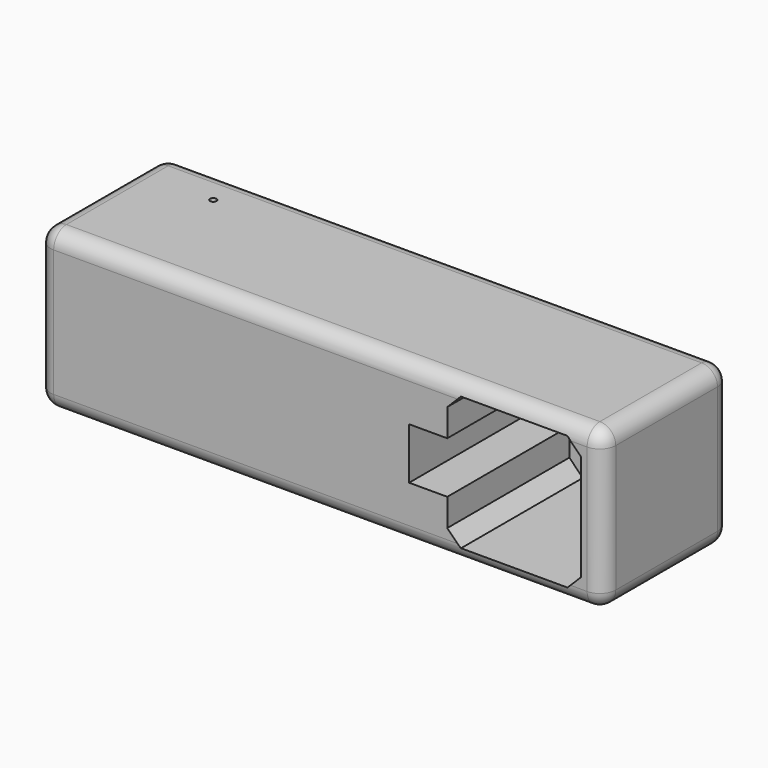
from build123d import *

# Parameters (mm, degrees)
F0_W           = 177.8
F0_H           = 50
F1_DEPTH       = 50
F2_W           = 12
F2_H           = 16.2
F3_DEPTH       = 50
F4_R           = 11
F5_DEPTH       = 5
F7_DEPTH       = 15
F8_R           = 0.49999
F9_T1_DEPTH    = 40
F9_T3_DEPTH    = 167.8
F9_T5_DEPTH    = 40
F9_S9_W        = 5
F9_S9_H        = 5
F9_T10_DEPTH   = 5
F9_S15_W       = 5
F9_S15_H       = 5
F9_T16_DEPTH   = 5
F9_S21_W       = 5
F9_S21_H       = 5
F9_T22_DEPTH   = 5
F9_S27_W       = 5
F9_S27_H       = 5
F9_T28_DEPTH   = 5
F9_S33_W       = 5
F9_S33_H       = 5
F9_T34_DEPTH   = 5
F9_S39_W       = 5
F9_S39_H       = 5
F9_T40_DEPTH   = 5
F9_S45_W       = 5
F9_S45_H       = 5
F9_T46_DEPTH   = 5
F9_S51_W       = 5
F9_S51_H       = 5
F9_T52_DEPTH   = 5
F10_R          = 1.6
F11_DEPTH      = 1
F12_R          = 1
F13_DEPTH      = 2
F13_DEPTH_BACK = 1
F14_DEPTH      = 25
F15_DEPTH      = 2
F16_R          = 11
F17_DEPTH      = 25


# Not quite as in the source:
# - a fillet or chamfer that OpenCascade refuses, or shapes differently, is made with other operations: its cross-section is extruded or revolved along the edge and cut away or added
# - a fillet or chamfer is up to 0.001 mm smaller than in the source, because OpenCascade refuses the exact size


with BuildPart() as f1:
    # F0 (on Front) → F1 (new body)
    with BuildSketch(Plane.XZ):
        Rectangle(F0_W, F0_H)
    extrude(amount=F1_DEPTH)

    # F2 (on face) → F3 (cut, through all)
    with BuildSketch(Plane(origin=(0, 0, 0), x_dir=(-1, 0, 0), z_dir=(0, 1, 0))):
        Polygon((-44.1426406871, 21), (-77.6573593129, 21), (-81.9, 16.7573593129), (-81.9, -16.7573593129), (-77.6573593129, -21), (-44.1426406871, -21), (-39.9, -16.7573593129), (-39.9, -8.1), (-39.9, 8.1), (-39.9, 16.7573593129), align=None)
        with BuildLine():
            ThreePointArc((-75, -15.6), (-77.5606601718, -16.6606601718), (-76.5, -14.1))
            Line((-76.5, -14.1), (-76.5, 14.1))
            ThreePointArc((-76.5, 14.1), (-77.5606601718, 16.6606601718), (-75, 15.6))
            Line((-75, 15.6), (-46.8, 15.6))
            ThreePointArc((-46.8, 15.6), (-45.3, 17.1), (-43.8, 15.6))
            ThreePointArc((-43.8, 15.6), (-44.2393398282, 14.5393398282), (-45.3, 14.1))
            Line((-45.3, 14.1), (-45.3, -14.1))
            ThreePointArc((-45.3, -14.1), (-44.2393398282, -14.5393398282), (-43.8, -15.6))
            ThreePointArc((-43.8, -15.6), (-45.3, -17.1), (-46.8, -15.6))
            Line((-46.8, -15.6), (-75, -15.6))
        make_face(mode=Mode.SUBTRACT)
        with Locations((-33.9, 0)):
            Rectangle(F2_W, F2_H)
        with BuildLine():
            Line((-75, -15.6), (-76.5, -15.6))
            Line((-76.5, -15.6), (-76.5, -14.1))
            ThreePointArc((-76.5, -14.1), (-77.5606601718, -16.6606601718), (-75, -15.6))
        make_face()
        with BuildLine():
            Line((-76.5, -14.1), (-76.5, -15.6))
            Line((-76.5, -15.6), (-75, -15.6))
            ThreePointArc((-75, -15.6), (-75.4393398282, -14.5393398282), (-76.5, -14.1))
        make_face()
        with BuildLine():
            Line((-76.5, 14.1), (-76.5, -14.1))
            ThreePointArc((-76.5, -14.1), (-75.4393398282, -14.5393398282), (-75, -15.6))
            Line((-75, -15.6), (-46.8, -15.6))
            ThreePointArc((-46.8, -15.6), (-46.3606601718, -14.5393398282), (-45.3, -14.1))
            Line((-45.3, -14.1), (-45.3, 14.1))
            ThreePointArc((-45.3, 14.1), (-46.3606601718, 14.5393398282), (-46.8, 15.6))
            Line((-46.8, 15.6), (-75, 15.6))
            ThreePointArc((-75, 15.6), (-75.4393398282, 14.5393398282), (-76.5, 14.1))
        make_face()
        with BuildLine():
            ThreePointArc((-75, 15.6), (-77.5606601718, 16.6606601718), (-76.5, 14.1))
            Line((-76.5, 14.1), (-76.5, 15.6))
            Line((-76.5, 15.6), (-75, 15.6))
        make_face()
        with BuildLine():
            Line((-76.5, 15.6), (-76.5, 14.1))
            ThreePointArc((-76.5, 14.1), (-75.4393398282, 14.5393398282), (-75, 15.6))
            Line((-75, 15.6), (-76.5, 15.6))
        make_face()
        with BuildLine():
            ThreePointArc((-45.3, -14.1), (-46.3606601718, -14.5393398282), (-46.8, -15.6))
            Line((-46.8, -15.6), (-45.3, -15.6))
            Line((-45.3, -15.6), (-45.3, -14.1))
        make_face()
        with BuildLine():
            Line((-45.3, -15.6), (-46.8, -15.6))
            ThreePointArc((-46.8, -15.6), (-45.3, -17.1), (-43.8, -15.6))
            ThreePointArc((-43.8, -15.6), (-44.2393398282, -14.5393398282), (-45.3, -14.1))
            Line((-45.3, -14.1), (-45.3, -15.6))
        make_face()
        with BuildLine():
            ThreePointArc((-43.8, 15.6), (-45.3, 17.1), (-46.8, 15.6))
            Line((-46.8, 15.6), (-45.3, 15.6))
            Line((-45.3, 15.6), (-45.3, 14.1))
            ThreePointArc((-45.3, 14.1), (-44.2393398282, 14.5393398282), (-43.8, 15.6))
        make_face()
        with BuildLine():
            Line((-45.3, 15.6), (-46.8, 15.6))
            ThreePointArc((-46.8, 15.6), (-46.3606601718, 14.5393398282), (-45.3, 14.1))
            Line((-45.3, 14.1), (-45.3, 15.6))
        make_face()
    extrude(amount=-F3_DEPTH, mode=Mode.SUBTRACT)

    # F4 (on face) → F5 (cut)
    with BuildSketch(Plane(origin=(0, 0, 0), x_dir=(-1, 0, 0), z_dir=(0, 1, 0))):
        with Locations((63.9, 0)):
            Circle(F4_R)
    extrude(amount=-F5_DEPTH, mode=Mode.SUBTRACT)

    # F6 (on face) → F7 (cut)
    with BuildSketch(Plane(origin=(0, -5, 0), x_dir=(-1, 0, 0), z_dir=(0, 1, 0))):
        with BuildLine():
            Line((65.4, 2), (62.4, 2))
            ThreePointArc((62.4, 2), (63.9, -2.5), (65.4, 2))
        make_face()
    extrude(amount=-F7_DEPTH, mode=Mode.SUBTRACT)

    # F8 (radius 0.5 in the source; OpenCascade refuses exactly that, so slightly less here)
    f8_edges = [f1.edges().sort_by_distance(p)[0] for p in [
        (-63.9, -20, -2.5),
    ]]
    fillet(f8_edges, radius=F8_R)

    # F9: fillet of radius 5 on 12 edges, made by hand

    # F9_s2 → F9_t1 (cut)
    with BuildSketch(Plane.XZ.offset(5)):
        with BuildLine():
            ThreePointArc((-88.9, 20), (-87.4355339059, 23.5355339059), (-83.9, 25))
            Line((-83.9, 25), (-88.9, 25))
            Line((-88.9, 25), (-88.9, 20))
        make_face()
        with BuildLine():
            ThreePointArc((83.9, 25), (87.4355339059, 23.5355339059), (88.9, 20))
            Line((88.9, 20), (88.9, 25))
            Line((88.9, 25), (83.9, 25))
        make_face()
        with BuildLine():
            ThreePointArc((-88.9, -20), (-87.4355339059, -23.5355339059), (-83.9, -25))
            Line((-83.9, -25), (-88.9, -25))
            Line((-88.9, -25), (-88.9, -20))
        make_face()
        with BuildLine():
            ThreePointArc((83.9, -25), (87.4355339059, -23.5355339059), (88.9, -20))
            Line((88.9, -20), (88.9, -25))
            Line((88.9, -25), (83.9, -25))
        make_face()
    extrude(amount=F9_T1_DEPTH, mode=Mode.SUBTRACT)

    # F9_s4 → F9_t3 (cut)
    with BuildSketch(Plane.YZ.offset(-83.9)):
        with BuildLine():
            ThreePointArc((-45, 25), (-48.5355339059, 23.5355339059), (-50, 20))
            Line((-50, 20), (-50, 25))
            Line((-50, 25), (-45, 25))
        make_face()
        with BuildLine():
            ThreePointArc((-45, -25), (-48.5355339059, -23.5355339059), (-50, -20))
            Line((-50, -20), (-50, -25))
            Line((-50, -25), (-45, -25))
        make_face()
        with BuildLine():
            ThreePointArc((0, 20), (-1.4644660941, 23.5355339059), (-5, 25))
            Line((-5, 25), (0, 25))
            Line((0, 25), (0, 20))
        make_face()
        with BuildLine():
            ThreePointArc((0, -20), (-1.4644660941, -23.5355339059), (-5, -25))
            Line((-5, -25), (0, -25))
            Line((0, -25), (0, -20))
        make_face()
    extrude(amount=F9_T3_DEPTH, mode=Mode.SUBTRACT)

    # F9_s6 → F9_t5 (cut)
    with BuildSketch(Plane.XY.offset(-20)):
        with BuildLine():
            ThreePointArc((88.9, -45), (87.4355339059, -48.5355339059), (83.9, -50))
            Line((83.9, -50), (88.9, -50))
            Line((88.9, -50), (88.9, -45))
        make_face()
        with BuildLine():
            ThreePointArc((83.9, 0), (87.4355339059, -1.4644660941), (88.9, -5))
            Line((88.9, -5), (88.9, 0))
            Line((88.9, 0), (83.9, 0))
        make_face()
        with BuildLine():
            ThreePointArc((-83.9, 0), (-87.4355339059, -1.4644660941), (-88.9, -5))
            Line((-88.9, -5), (-88.9, 0))
            Line((-88.9, 0), (-83.9, 0))
        make_face()
        with BuildLine():
            ThreePointArc((-88.9, -45), (-87.4355339059, -48.5355339059), (-83.9, -50))
            Line((-83.9, -50), (-88.9, -50))
            Line((-88.9, -50), (-88.9, -45))
        make_face()
    extrude(amount=F9_T5_DEPTH, mode=Mode.SUBTRACT)


with BuildPart() as f9_tool8:
    # F9_s9 → F9_t10 (new body)
    with BuildSketch(Plane.XY.offset(20)):
        with Locations((-86.4, -2.5)):
            Rectangle(F9_S9_W, F9_S9_H)
    extrude(amount=F9_T10_DEPTH)

    # F9_s11 → F9_t12 (revolve, cut)
    with BuildSketch(Plane(origin=(-83.9, -5, 20), x_dir=(0.7071067812, -0.7071067812, 0), z_dir=(-0.7071067812, -0.7071067812, 0))):
        with BuildLine():
            ThreePointArc((0, -5), (5, 0), (0, 5))
            Line((0, 5), (0, -5))
        make_face()
    revolve(axis=Axis((-83.9, -5, 20), (0, 0, 1)), mode=Mode.SUBTRACT)


with BuildPart() as f1_1:
    add(f1.part)

    # F9_t7: cut F9_tool8
    add(f9_tool8.part, mode=Mode.SUBTRACT)


with BuildPart() as f9_tool14:
    # F9_s15 → F9_t16 (new body)
    with BuildSketch(Plane.XY.offset(20)):
        with Locations((-86.4, -47.5)):
            Rectangle(F9_S15_W, F9_S15_H)
    extrude(amount=F9_T16_DEPTH)

    # F9_s17 → F9_t18 (revolve, cut)
    with BuildSketch(Plane(origin=(-83.9, -45, 20), x_dir=(0.7071067812, 0.7071067812, 0), z_dir=(0.7071067812, -0.7071067812, 0))):
        with BuildLine():
            ThreePointArc((0, -5), (5, 0), (0, 5))
            Line((0, 5), (0, -5))
        make_face()
    revolve(axis=Axis((-83.9, -45, 20), (0, 0, 1)), mode=Mode.SUBTRACT)


with BuildPart() as f1_2:
    add(f1_1.part)

    # F9_t13: cut F9_tool14
    add(f9_tool14.part, mode=Mode.SUBTRACT)


with BuildPart() as f9_tool20:
    # F9_s21 → F9_t22 (new body)
    with BuildSketch(Plane.XY.offset(20)):
        with Locations((86.4, -47.5)):
            Rectangle(F9_S21_W, F9_S21_H)
    extrude(amount=F9_T22_DEPTH)

    # F9_s23 → F9_t24 (revolve, cut)
    with BuildSketch(Plane(origin=(83.9, -45, 20), x_dir=(-0.7071067812, 0.7071067812, 0), z_dir=(0.7071067812, 0.7071067812, 0))):
        with BuildLine():
            ThreePointArc((0, -5), (5, 0), (0, 5))
            Line((0, 5), (0, -5))
        make_face()
    revolve(axis=Axis((83.9, -45, 20), (0, 0, 1)), mode=Mode.SUBTRACT)


with BuildPart() as f1_3:
    add(f1_2.part)

    # F9_t19: cut F9_tool20
    add(f9_tool20.part, mode=Mode.SUBTRACT)


with BuildPart() as f9_tool26:
    # F9_s27 → F9_t28 (new body)
    with BuildSketch(Plane.XY.offset(-20)):
        with Locations((-86.4, -47.5)):
            Rectangle(F9_S27_W, F9_S27_H)
    extrude(amount=-F9_T28_DEPTH)

    # F9_s29 → F9_t30 (revolve, cut)
    with BuildSketch(Plane(origin=(-83.9, -45, -20), x_dir=(0.7071067812, 0.7071067812, 0), z_dir=(-0.7071067812, 0.7071067812, 0))):
        with BuildLine():
            ThreePointArc((0, -5), (5, 0), (0, 5))
            Line((0, 5), (0, -5))
        make_face()
    revolve(axis=Axis((-83.9, -45, -20), (0, 0, -1)), mode=Mode.SUBTRACT)


with BuildPart() as f1_4:
    add(f1_3.part)

    # F9_t25: cut F9_tool26
    add(f9_tool26.part, mode=Mode.SUBTRACT)


with BuildPart() as f9_tool32:
    # F9_s33 → F9_t34 (new body)
    with BuildSketch(Plane.XY.offset(-20)):
        with Locations((86.4, -47.5)):
            Rectangle(F9_S33_W, F9_S33_H)
    extrude(amount=-F9_T34_DEPTH)

    # F9_s35 → F9_t36 (revolve, cut)
    with BuildSketch(Plane(origin=(83.9, -45, -20), x_dir=(-0.7071067812, 0.7071067812, 0), z_dir=(-0.7071067812, -0.7071067812, 0))):
        with BuildLine():
            ThreePointArc((0, -5), (5, 0), (0, 5))
            Line((0, 5), (0, -5))
        make_face()
    revolve(axis=Axis((83.9, -45, -20), (0, 0, -1)), mode=Mode.SUBTRACT)


with BuildPart() as f1_5:
    add(f1_4.part)

    # F9_t31: cut F9_tool32
    add(f9_tool32.part, mode=Mode.SUBTRACT)


with BuildPart() as f9_tool38:
    # F9_s39 → F9_t40 (new body)
    with BuildSketch(Plane.XY.offset(20)):
        with Locations((86.4, -2.5)):
            Rectangle(F9_S39_W, F9_S39_H)
    extrude(amount=F9_T40_DEPTH)

    # F9_s41 → F9_t42 (revolve, cut)
    with BuildSketch(Plane(origin=(83.9, -5, 20), x_dir=(-0.7071067812, -0.7071067812, 0), z_dir=(-0.7071067812, 0.7071067812, 0))):
        with BuildLine():
            ThreePointArc((0, -5), (5, 0), (0, 5))
            Line((0, 5), (0, -5))
        make_face()
    revolve(axis=Axis((83.9, -5, 20), (0, 0, 1)), mode=Mode.SUBTRACT)


with BuildPart() as f1_6:
    add(f1_5.part)

    # F9_t37: cut F9_tool38
    add(f9_tool38.part, mode=Mode.SUBTRACT)


with BuildPart() as f9_tool44:
    # F9_s45 → F9_t46 (new body)
    with BuildSketch(Plane.XY.offset(-20)):
        with Locations((86.4, -2.5)):
            Rectangle(F9_S45_W, F9_S45_H)
    extrude(amount=-F9_T46_DEPTH)

    # F9_s47 → F9_t48 (revolve, cut)
    with BuildSketch(Plane(origin=(83.9, -5, -20), x_dir=(-0.7071067812, -0.7071067812, 0), z_dir=(0.7071067812, -0.7071067812, 0))):
        with BuildLine():
            ThreePointArc((0, -5), (5, 0), (0, 5))
            Line((0, 5), (0, -5))
        make_face()
    revolve(axis=Axis((83.9, -5, -20), (0, 0, -1)), mode=Mode.SUBTRACT)


with BuildPart() as f1_7:
    add(f1_6.part)

    # F9_t43: cut F9_tool44
    add(f9_tool44.part, mode=Mode.SUBTRACT)


with BuildPart() as f9_tool50:
    # F9_s51 → F9_t52 (new body)
    with BuildSketch(Plane.XY.offset(-20)):
        with Locations((-86.4, -2.5)):
            Rectangle(F9_S51_W, F9_S51_H)
    extrude(amount=-F9_T52_DEPTH)

    # F9_s53 → F9_t54 (revolve, cut)
    with BuildSketch(Plane(origin=(-83.9, -5, -20), x_dir=(0.7071067812, -0.7071067812, 0), z_dir=(0.7071067812, 0.7071067812, 0))):
        with BuildLine():
            ThreePointArc((0, -5), (5, 0), (0, 5))
            Line((0, 5), (0, -5))
        make_face()
    revolve(axis=Axis((-83.9, -5, -20), (0, 0, -1)), mode=Mode.SUBTRACT)


with BuildPart() as f1_8:
    add(f1_7.part)

    # F9_t49: cut F9_tool50
    add(f9_tool50.part, mode=Mode.SUBTRACT)

    # F10 (on face) → F11 (cut)
    with BuildSketch(Plane(origin=(0, 0, 0), x_dir=(-1, 0, 0), z_dir=(0, 1, 0))):
        with Locations((16.4, 1.07)):
            Circle(F10_R)
        with Locations((-8.7923407305, 3.1555858932)):
            Circle(F10_R)
    extrude(amount=-F11_DEPTH, mode=Mode.SUBTRACT)

    # F12 (on face) → F13 (cut, two sides)
    with BuildSketch(Plane(origin=(0, 0, 2), x_dir=(1, 0, 0), z_dir=(0, 0, -1))) as f13_sk:
        Polygon((-61.9, 13.4047005384), (-63.9, 14.5594010768), (-65.9, 13.4047005384), (-65.9, 11.0952994616), (-63.9, 9.9405989232), (-61.9, 11.0952994616), align=None)
        with Locations((-63.9, 12.25)):
            Circle(F12_R, mode=Mode.SUBTRACT)
    extrude(amount=-F13_DEPTH, mode=Mode.SUBTRACT)
    extrude(f13_sk.sketch, amount=F13_DEPTH_BACK, mode=Mode.SUBTRACT)

    # F12 (on face) → F14 (cut)
    with BuildSketch(Plane(origin=(0, 0, 2), x_dir=(1, 0, 0), z_dir=(0, 0, -1))):
        with Locations((-63.9, 12.25)):
            Circle(F12_R)
    extrude(amount=-F14_DEPTH, mode=Mode.SUBTRACT)

    # F2 (on face) → F15 (join)
    with BuildSketch(Plane(origin=(0, 0, 0), x_dir=(-1, 0, 0), z_dir=(0, 1, 0))):
        Polygon((-44.1426406871, 21), (-77.6573593129, 21), (-81.9, 16.7573593129), (-81.9, -16.7573593129), (-77.6573593129, -21), (-44.1426406871, -21), (-39.9, -16.7573593129), (-39.9, -8.1), (-39.9, 8.1), (-39.9, 16.7573593129), align=None)
        with BuildLine():
            ThreePointArc((-75, -15.6), (-77.5606601718, -16.6606601718), (-76.5, -14.1))
            Line((-76.5, -14.1), (-76.5, 14.1))
            ThreePointArc((-76.5, 14.1), (-77.5606601718, 16.6606601718), (-75, 15.6))
            Line((-75, 15.6), (-46.8, 15.6))
            ThreePointArc((-46.8, 15.6), (-45.3, 17.1), (-43.8, 15.6))
            ThreePointArc((-43.8, 15.6), (-44.2393398282, 14.5393398282), (-45.3, 14.1))
            Line((-45.3, 14.1), (-45.3, -14.1))
            ThreePointArc((-45.3, -14.1), (-44.2393398282, -14.5393398282), (-43.8, -15.6))
            ThreePointArc((-43.8, -15.6), (-45.3, -17.1), (-46.8, -15.6))
            Line((-46.8, -15.6), (-75, -15.6))
        make_face(mode=Mode.SUBTRACT)
        with Locations((-33.9, 0)):
            Rectangle(F2_W, F2_H)
        with BuildLine():
            Line((-76.5, 14.1), (-76.5, -14.1))
            ThreePointArc((-76.5, -14.1), (-75.4393398282, -14.5393398282), (-75, -15.6))
            Line((-75, -15.6), (-46.8, -15.6))
            ThreePointArc((-46.8, -15.6), (-46.3606601718, -14.5393398282), (-45.3, -14.1))
            Line((-45.3, -14.1), (-45.3, 14.1))
            ThreePointArc((-45.3, 14.1), (-46.3606601718, 14.5393398282), (-46.8, 15.6))
            Line((-46.8, 15.6), (-75, 15.6))
            ThreePointArc((-75, 15.6), (-75.4393398282, 14.5393398282), (-76.5, 14.1))
        make_face()
    extrude(amount=-F15_DEPTH)

    # F16 (on face) → F17 (cut)
    with BuildSketch(Plane(origin=(0, 0, 0), x_dir=(-1, 0, 0), z_dir=(0, 1, 0))):
        with Locations((-60.9, 0)):
            Circle(F16_R)
    extrude(amount=-F17_DEPTH, mode=Mode.SUBTRACT)


solid = f1_8.part
